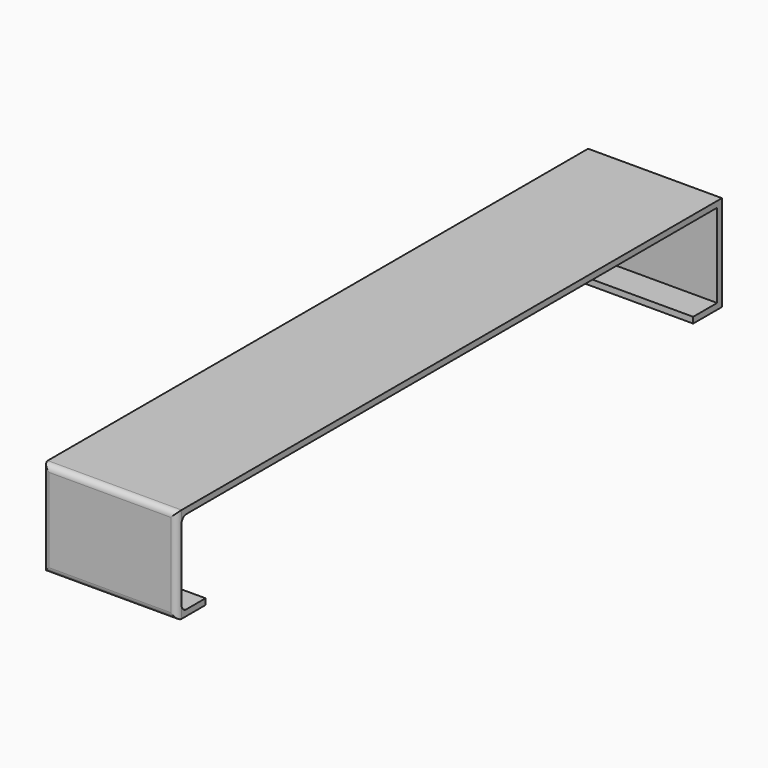
from build123d import *

# Parameters (mm, degrees)
F0_W     = 22.3398831487
F0_H     = 111.7630600929
F1_DEPTH = 1
F2_DEPTH = 1
F3_DEPTH = 1
F4_DEPTH = 14
F5_DEPTH = 14
F6_DEPTH = 1
F7_DEPTH = 1
F8_DEPTH = 5
F9_DEPTH = 5
F11_R    = 0.9999


# Not quite as in the source:
# - a fillet or chamfer is up to 0.001 mm smaller than in the source, because OpenCascade refuses the exact size


with BuildPart() as f1:
    # F0 (on Top) → F1 (new body)
    with BuildSketch(Plane.XY):
        with Locations((-9.3135908246, -6.8099498749)):
            Rectangle(F0_W, F0_H)
    extrude(amount=F1_DEPTH)


with BuildPart() as f2:
    # F2 (new): a face of the model
    f2_faces = [f1.part.faces().sort_by_distance(p)[0] for p in [
        (-9.3135908246, -62.6914799213, 0.5),
    ]]
    extrude(f2_faces, amount=F2_DEPTH)


with BuildPart() as f3:
    # F3 (new): a face of the model
    f3_faces = [f1.part.faces().sort_by_distance(p)[0] for p in [
        (-9.3135908246, 49.0715801716, 0.5),
    ]]
    extrude(f3_faces, amount=F3_DEPTH)


with BuildPart() as f4:
    # F4 (new): a face of the model
    f4_faces = [f3.part.faces().sort_by_distance(p)[0] for p in [
        (-9.3135908246, 49.5715801716, 0),
    ]]
    extrude(f4_faces, amount=F4_DEPTH)


with BuildPart() as f5:
    # F5 (new): a face of the model
    f5_faces = [f2.part.faces().sort_by_distance(p)[0] for p in [
        (-9.3135908246, -63.1914799213, 0),
    ]]
    extrude(f5_faces, amount=F5_DEPTH)


with BuildPart() as f6:
    # F6 (new): a face of the model
    f6_faces = [f5.part.faces().sort_by_distance(p)[0] for p in [
        (-9.3135908246, -63.1914799213, -14),
    ]]
    extrude(f6_faces, amount=F6_DEPTH)


with BuildPart() as f7:
    # F7 (new): a face of the model
    f7_faces = [f4.part.faces().sort_by_distance(p)[0] for p in [
        (-9.3135908246, 49.5715801716, -14),
    ]]
    extrude(f7_faces, amount=F7_DEPTH)


with BuildPart() as f8:
    # F8 (new): a face of the model
    f8_faces = [f6.part.faces().sort_by_distance(p)[0] for p in [
        (-9.3135908246, -62.6914799213, -14.5),
    ]]
    extrude(f8_faces, amount=F8_DEPTH)


with BuildPart() as f9:
    # F9 (new): a face of the model
    f9_faces = [f7.part.faces().sort_by_distance(p)[0] for p in [
        (-9.3135908246, 49.0715801716, -14.5),
    ]]
    extrude(f9_faces, amount=F9_DEPTH)


with BuildPart() as f8_1:
    add(f8.part)

    # F10: union F6, F5, F2, F1, F3, F4, F9, F7
    add(f6.part)
    add(f5.part)
    add(f2.part)
    add(f1.part)
    add(f3.part)
    add(f4.part)
    add(f9.part)
    add(f7.part)

    # F11 (radius 1 in the source; OpenCascade refuses exactly that, so slightly less here)
    f11_edges = [f8_1.edges().sort_by_distance(p)[0] for p in [
        (-9.313591, -62.69148, 0),
        (-20.483532, -63.69148, -7),
        (-9.313591, -63.69148, -15),
        (1.856351, -63.69148, -7),
        (-9.313591, -63.69148, 1),
        (-9.313591, -62.69148, -14),
    ]]
    fillet(f11_edges, radius=F11_R)


solid = f8_1.part
